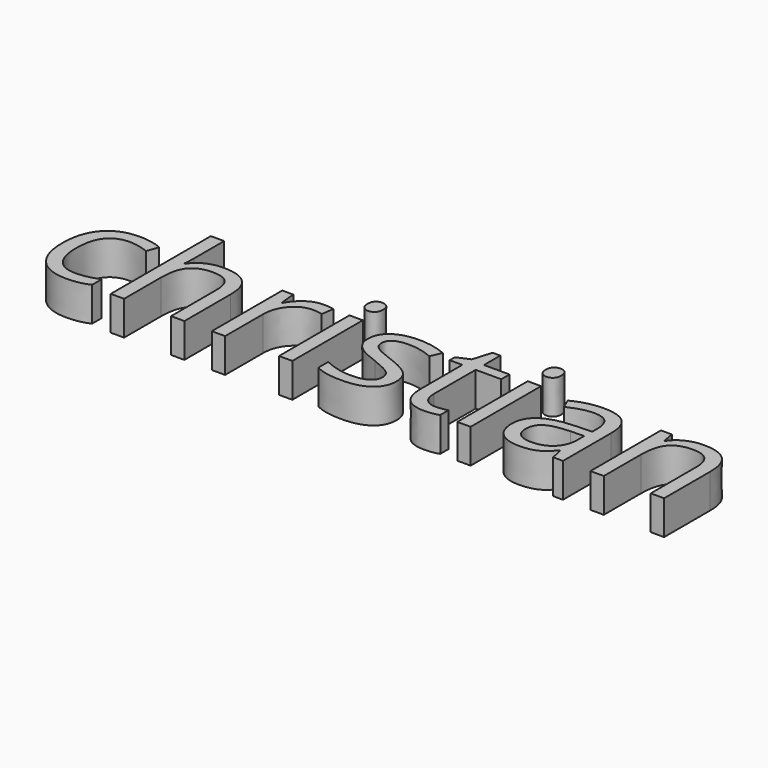
from build123d import *

# Parameters (mm, degrees)
F0_TEXT_SIZE = 120.3153282404
F1_DEPTH     = 25


# Not quite as in the source:
# - Text() gives the source's letters only with a copy of the font that has no kerning and outlines rounded to 1/6400 em; it was checked with that copy


with BuildPart() as f1:
    # F0 (on Top) → F1 (new body)
    with BuildSketch(Plane.XY):
        with Locations((-129.0799379349, -71.2825208902)):
            Text('christian', F0_TEXT_SIZE, font='Open Sans', text_align=(TextAlign.LEFT, TextAlign.BOTTOM))
    extrude(amount=F1_DEPTH)


solid = f1.part
